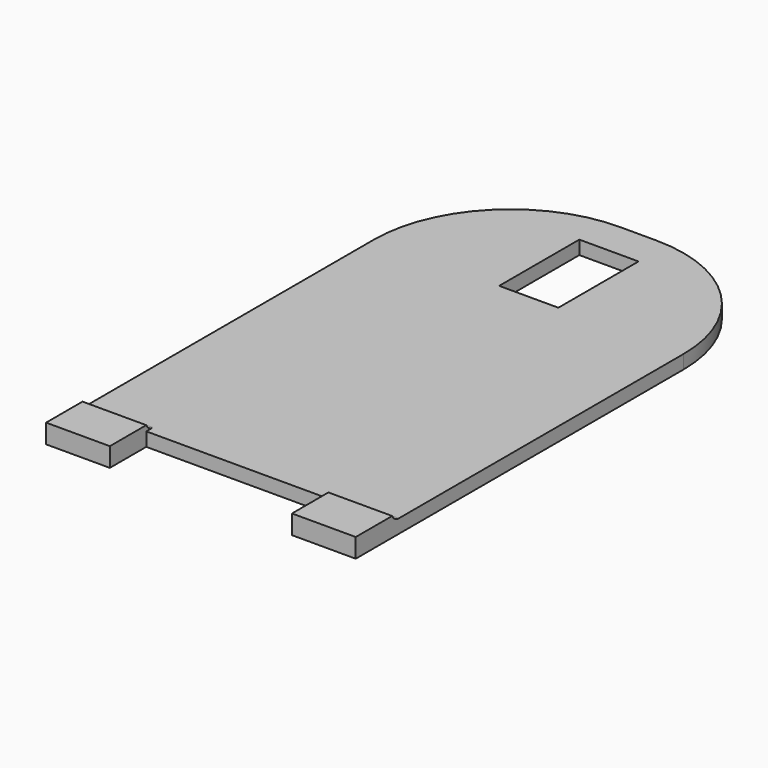
from build123d import *

# Parameters (mm, degrees)
F0_W        = 7
F0_H        = 5
F1_DEPTH    = 1.5
F2_R        = 15
F3_DEPTH    = 2.1
F4_T1_DEPTH = 7
F4_T3_DEPTH = 7


# Not quite as in the source:
# - a fillet or chamfer that OpenCascade refuses, or shapes differently, is made with other operations: its cross-section is extruded or revolved along the edge and cut away or added


with BuildPart() as f1:
    # F0 (on Top) → F1 (new body)
    with BuildSketch(Plane.XY):
        Polygon((0, 8.4325535595), (-17, 8.4325535595), (-17, -46.5674464405), (-10, -46.5674464405), (0, -46.5674464405), (0, -6.5674464405), (-3.25, -6.5674464405), (-3.25, 4.4325535595), (0, 4.4325535595), align=None)
        Polygon((17, 8.4325535595), (0, 8.4325535595), (0, 4.4325535595), (3.25, 4.4325535595), (3.25, -6.5674464405), (0, -6.5674464405), (0, -46.5674464405), (10, -46.5674464405), (17, -46.5674464405), align=None)
        with Locations((13.5, -49.0674464405)):
            Rectangle(F0_W, F0_H)
        with Locations((-13.5, -49.0674464405)):
            Rectangle(F0_W, F0_H)
    extrude(amount=F1_DEPTH)

    # F2
    f2_edges = [f1.edges().sort_by_distance(p)[0] for p in [
        (17, 8.432554, 0.75),
        (-17, 8.432554, 0.75),
    ]]
    fillet(f2_edges, radius=F2_R)

    # F0 (on Top) → F3 (join)
    with BuildSketch(Plane.XY):
        with Locations((13.5, -49.0674464405)):
            Rectangle(F0_W, F0_H)
        with Locations((-13.5, -49.0674464405)):
            Rectangle(F0_W, F0_H)
    extrude(amount=F3_DEPTH)

    # F4: fillet of radius 1 on 2 edges, made by hand

    # F4_s2 → F4_t1 (join)
    with BuildSketch(Plane.YZ.offset(-17)):
        with BuildLine():
            ThreePointArc((-46.5674464405, 2.1), (-46.198653859, 1.6633399735), (-45.6509313015, 1.5))
            Line((-45.6509313015, 1.5), (-46.5674464405, 1.5))
            Line((-46.5674464405, 1.5), (-46.5674464405, 2.1))
        make_face()
    extrude(amount=F4_T1_DEPTH)

    # F4_s4 → F4_t3 (join)
    with BuildSketch(Plane.YZ.offset(10)):
        with BuildLine():
            ThreePointArc((-46.5674464405, 2.1), (-46.198653859, 1.6633399735), (-45.6509313015, 1.5))
            Line((-45.6509313015, 1.5), (-46.5674464405, 1.5))
            Line((-46.5674464405, 1.5), (-46.5674464405, 2.1))
        make_face()
    extrude(amount=F4_T3_DEPTH)


solid = f1.part
